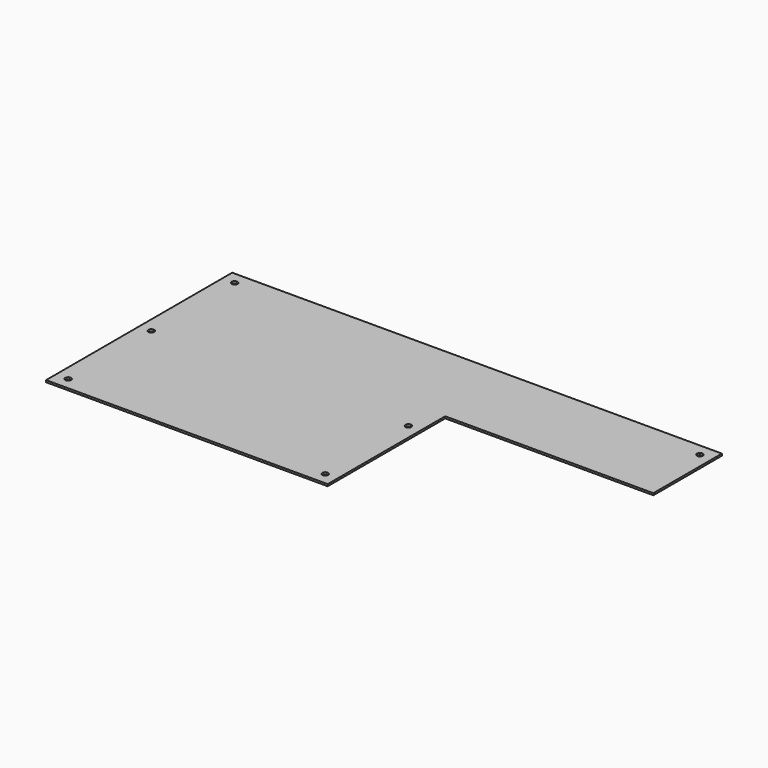
from build123d import *

# Parameters (mm, degrees)
F1_DEPTH = 1
F3_D     = 3.048
F3_DEPTH = 12.7
F3_TIP   = 0.9157115834


# Not quite as in the source:
# - a feature names something its author has since deleted; it is built from what else it names


with BuildPart() as f1:
    # F0 (on Top) → F1 (new body)
    with BuildSketch(Plane.XY):
        Polygon((127, 56.1535057819), (-127, 56.1535057819), (-127, 11.7035057819), (-127, -64.4964942181), (19.05, -64.4964942181), (19.05, 11.7035057819), (127, 11.7035057819), align=None)
    extrude(amount=F1_DEPTH)

    # F3
    with Locations(Plane.XY.offset(1)):
        with Locations((-120.65, 49.8035057819), (-120.65, -4.1714942181), (-120.65, -58.1464942181), (12.7, -58.1464942181), (12.7, -4.1714942181), (120.65, 49.8035057819)):
            Hole(F3_D / 2, depth=F3_DEPTH)
            with Locations((0, 0, -(F3_DEPTH + F3_TIP / 2))):  # 118° drill point
                Cone(0, F3_D / 2, F3_TIP, mode=Mode.SUBTRACT)


solid = f1.part
